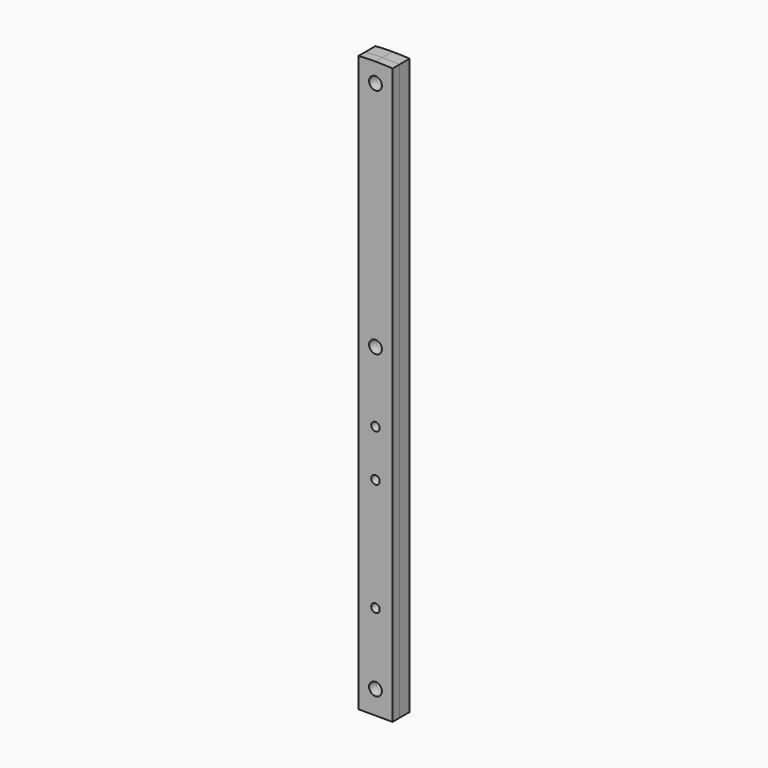
from build123d import *

# Parameters (mm, degrees)
F0_W     = 8
F0_H     = 9.6326530612
F0_R     = 1.5
F0_R_2   = 1
F1_DEPTH = 5
F2_DEPTH = 3


# Not quite as in the source:
# - a feature names something its author has since deleted; it is built from what else it names


with BuildPart() as f1:
    # F0 (on Front) → F1 (new body)
    with BuildSketch(Plane.XZ):
        with BuildLine():
            Line((-0.072881, 79.2495112755), (-0.072881, 33.2229425306))
            Line((-0.072881, 33.2229425306), (7.927119, 33.2229425306))
            Line((7.927119, 33.2229425306), (7.927119, 79.2495112755))
            ThreePointArc((7.927119, 79.2495112755), (3.927119, 79.406616), (-0.072881, 79.2495112755))
        make_face()
        with Locations((3.927119, 28.406616)):
            Rectangle(F0_W, F0_H)
        with Locations((3.927119, 28.406616)):
            Circle(F0_R, mode=Mode.SUBTRACT)
        with BuildLine():
            Line((7.927119, 23.5902894694), (-0.072881, 23.5902894694))
            Line((-0.072881, 23.5902894694), (-0.072881, -22.4362792755))
            ThreePointArc((-0.072881, -22.4362792755), (3.927119, -22.593384), (7.927119, -22.4362792755))
            Line((7.927119, -22.4362792755), (7.927119, 23.5902894694))
        make_face()
        with Locations((3.927119, 0.906616)):
            Circle(F0_R_2, mode=Mode.SUBTRACT)
        with Locations((3.927119, 11.906616)):
            Circle(F0_R_2, mode=Mode.SUBTRACT)
        with BuildLine():
            Line((-0.072881, 87.270866611), (-0.072881, 79.2495112755))
            ThreePointArc((-0.072881, 79.2495112755), (3.927119, 79.406616), (7.927119, 79.2495112755))
            Line((7.927119, 79.2495112755), (7.927119, 87.270866611))
            ThreePointArc((7.927119, 87.270866611), (5.9282704121, 87.3726688866), (3.927119, 87.406616))
            ThreePointArc((3.927119, 87.406616), (1.9259675879, 87.3726688866), (-0.072881, 87.270866611))
        make_face()
        with Locations((3.927119, 82.906616)):
            Circle(F0_R, mode=Mode.SUBTRACT)
        with BuildLine():
            ThreePointArc((7.927119, -22.4362792755), (3.927119, -22.593384), (-0.072881, -22.4362792755))
            Line((-0.072881, -22.4362792755), (-0.072881, -30.457634611))
            ThreePointArc((-0.072881, -30.457634611), (3.927119, -30.593384), (7.927119, -30.457634611))
            Line((7.927119, -30.457634611), (7.927119, -22.4362792755))
        make_face()
        with Locations((3.927119, -25.593384)):
            Circle(F0_R_2, mode=Mode.SUBTRACT)
        with BuildLine():
            ThreePointArc((7.927119, -30.457634611), (3.927119, -30.593384), (-0.072881, -30.457634611))
            Line((-0.072881, -30.457634611), (-0.072881, -47.833384))
            Line((-0.072881, -47.833384), (7.927119, -47.833384))
            Line((7.927119, -47.833384), (7.927119, -30.457634611))
        make_face()
        with Locations((3.927119, -42.333384)):
            Circle(F0_R, mode=Mode.SUBTRACT)
    extrude(amount=F1_DEPTH)


with BuildPart() as f2:
    # F0 (on Front) → F2 (new body)
    with BuildSketch(Plane.XZ):
        with BuildLine():
            Line((7.927119, 23.5902894694), (-0.072881, 23.5902894694))
            Line((-0.072881, 23.5902894694), (-0.072881, -22.4362792755))
            ThreePointArc((-0.072881, -22.4362792755), (3.927119, -22.593384), (7.927119, -22.4362792755))
            Line((7.927119, -22.4362792755), (7.927119, 23.5902894694))
        make_face()
        with Locations((3.927119, 0.906616)):
            Circle(F0_R_2, mode=Mode.SUBTRACT)
        with Locations((3.927119, 11.906616)):
            Circle(F0_R_2, mode=Mode.SUBTRACT)
        with BuildLine():
            ThreePointArc((7.927119, -22.4362792755), (3.927119, -22.593384), (-0.072881, -22.4362792755))
            Line((-0.072881, -22.4362792755), (-0.072881, -30.457634611))
            ThreePointArc((-0.072881, -30.457634611), (3.927119, -30.593384), (7.927119, -30.457634611))
            Line((7.927119, -30.457634611), (7.927119, -22.4362792755))
        make_face()
        with Locations((3.927119, -25.593384)):
            Circle(F0_R_2, mode=Mode.SUBTRACT)
        with BuildLine():
            ThreePointArc((7.927119, -30.457634611), (3.927119, -30.593384), (-0.072881, -30.457634611))
            Line((-0.072881, -30.457634611), (-0.072881, -47.833384))
            Line((-0.072881, -47.833384), (7.927119, -47.833384))
            Line((7.927119, -47.833384), (7.927119, -30.457634611))
        make_face()
        with Locations((3.927119, -42.333384)):
            Circle(F0_R, mode=Mode.SUBTRACT)
        with Locations((3.927119, 28.406616)):
            Rectangle(F0_W, F0_H)
        with Locations((3.927119, 28.406616)):
            Circle(F0_R, mode=Mode.SUBTRACT)
        with BuildLine():
            Line((-0.072881, 79.2495112755), (-0.072881, 33.2229425306))
            Line((-0.072881, 33.2229425306), (7.927119, 33.2229425306))
            Line((7.927119, 33.2229425306), (7.927119, 79.2495112755))
            ThreePointArc((7.927119, 79.2495112755), (3.927119, 79.406616), (-0.072881, 79.2495112755))
        make_face()
        with BuildLine():
            Line((-0.072881, 87.270866611), (-0.072881, 79.2495112755))
            ThreePointArc((-0.072881, 79.2495112755), (3.927119, 79.406616), (7.927119, 79.2495112755))
            Line((7.927119, 79.2495112755), (7.927119, 87.270866611))
            ThreePointArc((7.927119, 87.270866611), (5.9282704121, 87.3726688866), (3.927119, 87.406616))
            ThreePointArc((3.927119, 87.406616), (1.9259675879, 87.3726688866), (-0.072881, 87.270866611))
        make_face()
        with Locations((3.927119, 82.906616)):
            Circle(F0_R, mode=Mode.SUBTRACT)
    extrude(amount=F2_DEPTH)


solid = Compound([f1.part, f2.part])
